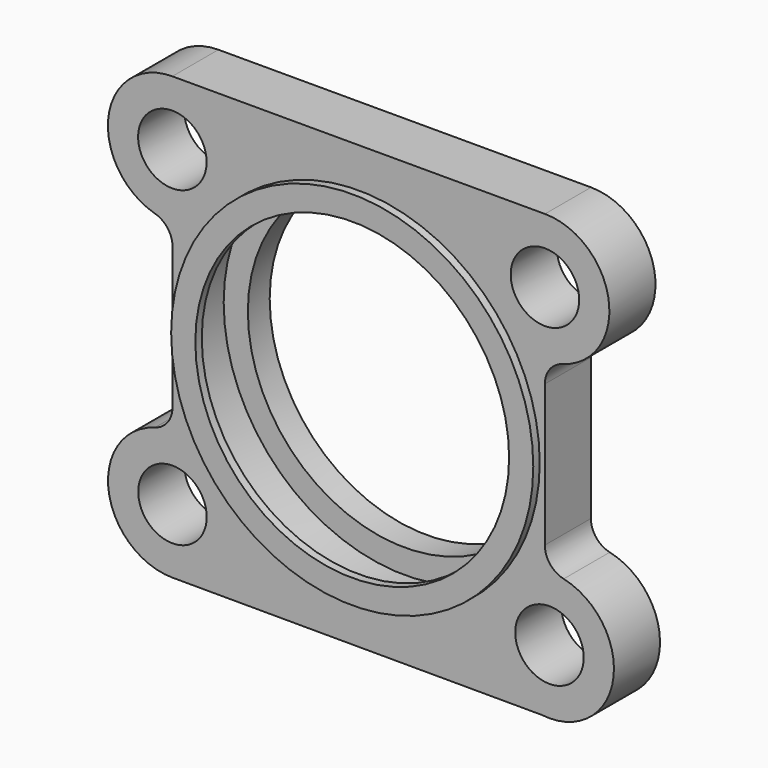
from build123d import *

# Parameters (mm, degrees)
F0_R     = 8.5
F0_R_2   = 44.95
F1_DEPTH = 14.3
F0_R_3   = 38.95
F2_DEPTH = 8.4
F3_R     = 44.95
F3_R_2   = 38.95
F4_DEPTH = 2


# Not quite as in the source:
# - a fillet or chamfer that OpenCascade refuses, or shapes differently, is made with other operations: its cross-section is extruded or revolved along the edge and cut away or added


with BuildPart() as f1:
    # F0 (on Front) → F1 (new body)
    with BuildSketch(Plane.XZ):
        with BuildLine():
            Line((-31.2142073288, 60.4033983739), (-123.7142073288, 60.4033983739))
            ThreePointArc((-123.7142073288, 60.4033983739), (-139.5634042419, 46.5949633879), (-128.0560255107, 29.0037680252))
            ThreePointArc((-128.0560255107, 29.0037680252), (-124.9004279177, 26.8504331935), (-123.6842073288, 23.2289066444))
            Line((-123.6842073288, 23.2289066444), (-123.6842073288, -11.9910933556))
            ThreePointArc((-123.6842073288, -11.9910933556), (-124.8978631175, -15.6092294905), (-128.0478436925, -17.7636416706))
            ThreePointArc((-128.0478436925, -17.7636416706), (-139.5318474493, -35.3598981178), (-123.6842073288, -49.1571038441))
            Line((-123.6842073288, -49.1571038441), (-31.9460769585, -49.3417102723))
            ThreePointArc((-31.9460769585, -49.3417102723), (-14.3192733633, -36.1434315621), (-26.5660258966, -17.8427261582))
            ThreePointArc((-26.5660258966, -17.8427261582), (-29.9309392076, -15.7364080757), (-31.2442073288, -11.9901373572))
            Line((-31.2442073288, -11.9901373572), (-31.2442073288, 23.2298626428))
            ThreePointArc((-31.2442073288, 23.2298626428), (-30.0282764979, 26.8510064104), (-26.873313267, 29.0044633946))
            ThreePointArc((-26.873313267, 29.0044633946), (-15.3683421549, 46.5945536538), (-31.2142073288, 60.4033983739))
        make_face()
        with Locations((-123.6842073288, -33.1571038441)):
            Circle(F0_R, mode=Mode.SUBTRACT)
        with Locations((-30.0908754106, -33.4496296276)):
            Circle(F0_R, mode=Mode.SUBTRACT)
        with Locations((-77.4642073288, 5.5766425614)):
            Circle(F0_R_2, mode=Mode.SUBTRACT)
        with Locations((-123.7142073288, 44.4033983739)):
            Circle(F0_R, mode=Mode.SUBTRACT)
        with Locations((-31.2175957686, 44.4033987327)):
            Circle(F0_R, mode=Mode.SUBTRACT)
    extrude(amount=F1_DEPTH)

    # F0 (on Front) → F2 (join)
    with BuildSketch(Plane.XZ):
        with Locations((-77.4642073288, 5.5766425614)):
            Circle(F0_R_2)
        with Locations((-77.4642073288, 5.5766425614)):
            Circle(F0_R_3, mode=Mode.SUBTRACT)
    extrude(amount=-F2_DEPTH)

    # F5: chamfer of 7.62 on 1 edges, made by hand

    # F5_s1 → F5_t2 (revolve, cut)
    with BuildSketch(Plane.XY.offset(5.5766425614)):
        Polygon((-32.5142073288, 0.78), (-40.1342073288, 8.4), (-32.5142073288, 8.4), align=None)
    revolve(axis=Axis((-77.4642073288, 8.4, 5.5766425614), (0, -1, 0)), mode=Mode.SUBTRACT)


with BuildPart() as f4:
    # F3 (on face) → F4 (new body)
    with BuildSketch(Plane.XZ.offset(14.3)):
        with Locations((-77.4642073288, 5.5766425614)):
            Circle(F3_R)
        with Locations((-77.4642073288, 5.5766425614)):
            Circle(F3_R_2, mode=Mode.SUBTRACT)
    extrude(amount=F4_DEPTH)


solid = Compound([f1.part, f4.part])
